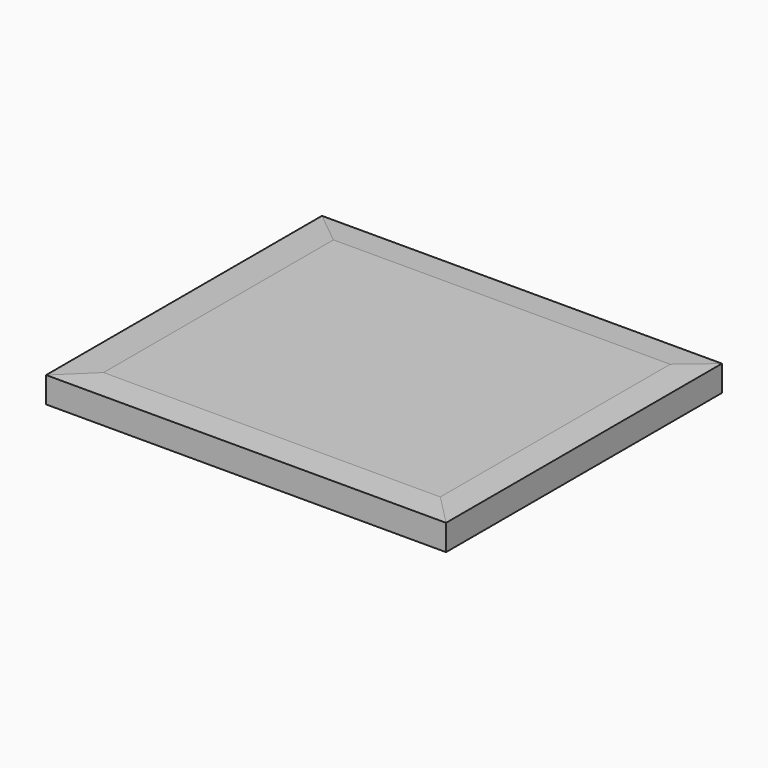
from build123d import *

# Parameters (mm, degrees)
F0_W        = 17678.4
F0_H        = 15240
F1_DEPTH    = 1219.2
F3_DEPTH    = 15240.001
F4_T1_DEPTH = 22757.9615534728
F4_T3_DEPTH = 21843.5615534728


# Not quite as in the source:
# - a fillet or chamfer that OpenCascade refuses, or shapes differently, is made with other operations: its cross-section is extruded or revolved along the edge and cut away or added


with BuildPart() as f1:
    # F0 (on Top) → F1 (new body)
    with BuildSketch(Plane.XY):
        with Locations((8839.2, 7620)):
            Rectangle(F0_W, F0_H)
    extrude(amount=F1_DEPTH)

    # F2 (on face) → F3 (cut, through all)
    with BuildSketch(Plane.XZ):
        Polygon((0, 1219.2), (0, 1143), (1524, 1219.2), align=None)
    extrude(amount=-F3_DEPTH, mode=Mode.SUBTRACT)

    # F4: chamfer of 1270 x 76.2 on 3 edges, made by hand

    # F4_s2 → F4_t1 (cut)
    with BuildSketch(Plane.YZ.offset(-1777.7807767364)):
        Polygon((1270, 1219.2), (0, 1143), (0, 1219.2), align=None)
        Polygon((15240, 1143), (13970, 1219.2), (15240, 1219.2), align=None)
    extrude(amount=F4_T1_DEPTH, mode=Mode.SUBTRACT)

    # F4_s4 → F4_t3 (cut)
    with BuildSketch(Plane.XZ.offset(-18541.7807767364)):
        Polygon((16408.4, 1219.2), (17678.4, 1143), (17678.4, 1219.2), align=None)
    extrude(amount=F4_T3_DEPTH, mode=Mode.SUBTRACT)


solid = f1.part
